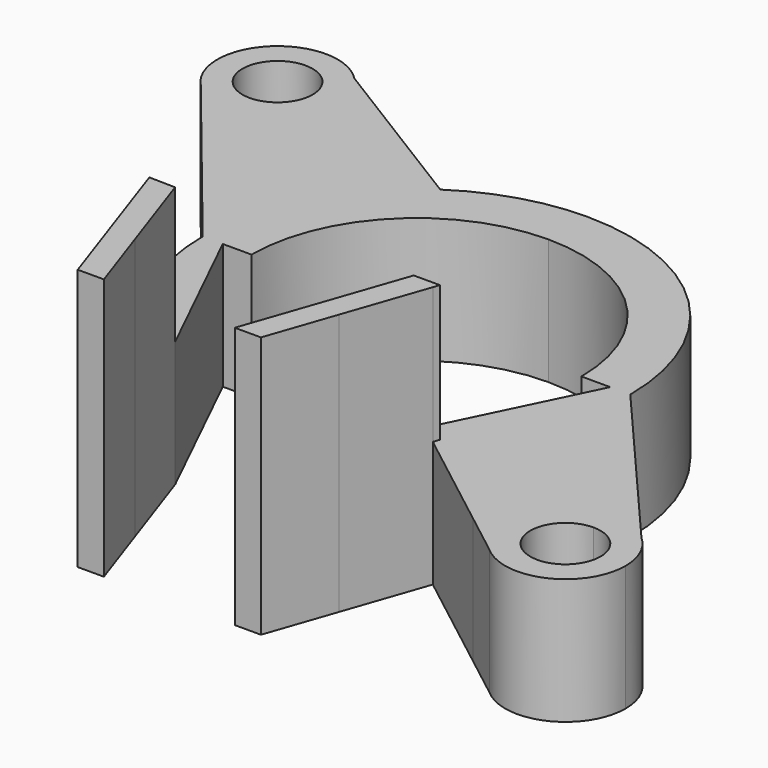
from build123d import *

# Parameters (mm, degrees)
F1_DEPTH = 12
F2_DEPTH = 25


# Not quite as in the source:
# - ends of sketch curves that miss each other by under 0.0002 mm in the source are joined


with BuildPart() as f1:
    # F0 (on Top) → F1 (new body)
    with BuildSketch(Plane.XY):
        with BuildLine():
            Line((-45.2079510631, 38.1848650801), (-50.0674114416, 38.1848649627))
            ThreePointArc((-50.0674114416, 38.1848649627), (-51.7515474497, 34.119000832), (-55.8174114415, 32.4348648238))
            Line((-55.8174114415, 32.4348648238), (-55.8174114414, 29.083605512))
            Line((-55.8174114414, 29.083605512), (-44.5532578407, 15.1687110318))
            ThreePointArc((-44.5532578407, 15.1687110318), (-42.1350647352, 24.8048651036), (-35.4555304308, 32.1592477879))
            Line((-35.4555304308, 32.1592477879), (-45.2079510631, 38.1848650801))
        make_face()
        with BuildLine():
            Line((-50.0674114416, 38.1848649627), (-52.4674114416, 38.1848649047))
            ThreePointArc((-52.4674114416, 38.1848649047), (-53.4486037246, 35.8160571069), (-55.8174114415, 34.8348648238))
            Line((-55.8174114415, 34.8348648238), (-55.8174114415, 32.4348648238))
            ThreePointArc((-55.8174114415, 32.4348648238), (-51.7515474497, 34.119000832), (-50.0674114416, 38.1848649627))
        make_face()
        with BuildLine():
            Line((-55.8174114414, 29.083605512), (-55.8174114415, 32.4348648238))
            ThreePointArc((-55.8174114415, 32.4348648238), (-58.0556968865, 32.8883963526), (-59.9408925855, 34.1774462962))
            Line((-59.9408925855, 34.1774462962), (-55.8174114414, 29.083605512))
        make_face()
        with BuildLine():
            Line((-55.8174114415, 32.4348648238), (-55.8174114415, 34.8348648238))
            ThreePointArc((-55.8174114415, 34.8348648238), (-57.1214560051, 35.0990962362), (-58.2197874124, 35.8501079425))
            Line((-58.2197874124, 35.8501079425), (-59.9408925855, 34.1774462962))
            ThreePointArc((-59.9408925855, 34.1774462962), (-58.0556968865, 32.8883963526), (-55.8174114415, 32.4348648238))
        make_face()
        with BuildLine():
            ThreePointArc((-58.2197874124, 35.8501079425), (-58.1521683229, 40.5872407946), (-53.4150354708, 40.5196217052))
            Line((-53.4150354708, 40.5196217052), (-51.6939302977, 42.1922833515))
            ThreePointArc((-51.6939302977, 42.1922833515), (-59.8248299692, 42.3083459677), (-59.9408925855, 34.1774462962))
            Line((-59.9408925855, 34.1774462962), (-58.2197874124, 35.8501079425))
        make_face()
        with BuildLine():
            ThreePointArc((-53.4150354708, 40.5196217052), (-52.7133447942, 39.4447339634), (-52.4674114416, 38.1848648238))
            Line((-52.4674114416, 38.1848648238), (-50.0674114416, 38.1848649627))
            ThreePointArc((-50.0674114416, 38.1848649627), (-50.4895358529, 40.3473267799), (-51.6939302977, 42.1922833515))
            Line((-51.6939302977, 42.1922833515), (-53.4150354708, 40.5196217052))
        make_face()
        with BuildLine():
            ThreePointArc((-51.6939302977, 42.1922833515), (-50.4895358529, 40.3473267799), (-50.0674114416, 38.1848648238))
            Line((-50.0674114416, 38.1848648238), (-45.2079510631, 38.1848650801))
            Line((-45.2079510631, 38.1848650801), (-51.6939302977, 42.1922833515))
        make_face()
        with BuildLine():
            ThreePointArc((-24.1338443596, 35.5853722206), (-30.0482104313, 34.7100811604), (-35.4555304308, 32.1592477879))
            ThreePointArc((-35.4555304308, 32.1592477879), (-42.1350647352, 24.8048651036), (-44.5532578407, 15.1687110318))
            Line((-44.5532578407, 15.1687110318), (-42.6338443592, 15.1659585535))
            Line((-42.6338443592, 15.1659585535), (-39.8838443592, 15.1659585535))
            ThreePointArc((-39.8838443592, 15.1659585535), (-35.270776163, 26.3028903571), (-24.1338443595, 30.9159585535))
            Line((-24.1338443595, 30.9159585535), (-24.1338443596, 35.5853722206))
        make_face()
        with BuildLine():
            ThreePointArc((-3.7144306922, 15.1659585535), (-9.6951384875, 29.6046644255), (-24.1338443596, 35.5853722206))
            Line((-24.1338443596, 35.5853722206), (-24.1338443595, 30.9159585535))
            ThreePointArc((-24.1338443595, 30.9159585535), (-12.9969125556, 26.3028903573), (-8.3838443592, 15.1659585535))
            Line((-8.3838443592, 15.1659585535), (-5.6338443592, 15.1659585535))
            Line((-5.6338443592, 15.1659585535), (-3.7144306922, 15.1659585535))
        make_face()
        with BuildLine():
            Line((-42.6338443592, 15.1659585535), (-44.5532578407, 15.1687110318))
            ThreePointArc((-44.5532578407, 15.1687110318), (-42.7914410163, 6.8685769492), (-37.807970261, 0.0011725238))
            Line((-37.807970261, 0.0011725238), (-38.0284454354, 0.643162408))
            Line((-38.0284454354, 0.643162408), (-35.5289696075, 0.5919707473))
            Line((-35.5289696075, 0.5919707473), (-42.6338443592, 15.1659585535))
        make_face()
        Polygon((-38.0284454354, 0.643162408), (-37.807970261, 0.0011725238), (-35.1236572441, -7.8151351762), (-32.6315665225, -7.8151351762), (-35.5289696075, 0.5919707473), align=None)
        Polygon((-32.6315665225, -7.8151351762), (-35.1236572441, -7.8151351762), (-32.8838443592, -14.3371266833), (-30.3838443592, -14.3371266833), align=None)
        Polygon((-13.136122196, -7.8151351762), (-15.636122196, -7.8151351762), (-17.8838443592, -14.3371266833), (-15.3838443592, -14.3371266833), align=None)
        Polygon((-10.2387191109, 0.5919707473), (-12.7387191109, 0.5919707473), (-15.636122196, -7.8151351762), (-13.136122196, -7.8151351762), (-10.4427343672, 0), align=None)
        with BuildLine():
            Line((7.5497227229, 2.079326472), (-3.7144306922, 15.1659585535))
            Line((-3.7144306922, 15.1659585535), (-5.6338443592, 15.1659585535))
            Line((-5.6338443592, 15.1659585535), (-12.7387191109, 0.5919707473))
            Line((-12.7387191109, 0.5919707473), (-10.2387191109, 0.5919707473))
            Line((-10.2387191109, 0.5919707473), (-10.4427343672, 0))
            Line((-10.4427343672, 0), (-0.3331204375, -7.8151351762))
            Line((-0.3331204375, -7.8151351762), (1.9170354556, -7.8151351762))
            ThreePointArc((1.9170354556, -7.8151351762), (3.0939956275, -3.0251503303), (7.549722723, -0.909568585))
            Line((7.549722723, -0.909568585), (7.5497227229, 2.079326472))
        make_face()
        with BuildLine():
            ThreePointArc((13.2997227231, -6.659568585), (12.7982725871, -4.3111171112), (11.3813838275, -2.3722765282))
            Line((11.3813838275, -2.3722765282), (9.7820818013, -4.1617549519))
            ThreePointArc((9.7820818013, -4.1617549519), (10.6075735134, -5.2913403351), (10.8997227231, -6.659568585))
            ThreePointArc((10.8997227231, -6.659568585), (8.917950973, -9.7174193754), (5.3173636448, -9.1573822181))
            Line((5.3173636448, -9.1573822181), (3.7180616186, -10.9468606418))
            ThreePointArc((3.7180616186, -10.9468606418), (9.8981741968, -11.908118449), (13.2997227231, -6.659568585))
        make_face()
        with BuildLine():
            ThreePointArc((11.3813838275, -2.3722765282), (9.6004019609, -1.2876774223), (7.549722723, -0.909568585))
            Line((7.549722723, -0.909568585), (7.549722723, -3.309568585))
            ThreePointArc((7.549722723, -3.309568585), (8.744466279, -3.5298580815), (9.7820818013, -4.1617549519))
            Line((9.7820818013, -4.1617549519), (11.3813838275, -2.3722765282))
        make_face()
        with BuildLine():
            Line((7.549722723, -3.309568585), (7.549722723, -0.909568585))
            ThreePointArc((7.549722723, -0.909568585), (3.0939956275, -3.0251503303), (1.9170354556, -7.8151351762))
            ThreePointArc((1.9170354556, -7.8151351762), (2.5652068364, -9.5261172721), (3.7180616186, -10.9468606418))
            Line((3.7180616186, -10.9468606418), (5.3173636448, -9.1573822181))
            ThreePointArc((5.3173636448, -9.1573822181), (4.4200122196, -5.464825029), (7.549722723, -3.309568585))
        make_face()
        with BuildLine():
            ThreePointArc((3.7180616186, -10.9468606418), (2.5652068364, -9.5261172721), (1.9170354556, -7.8151351762))
            Line((1.9170354556, -7.8151351762), (-0.3331204375, -7.8151351762))
            Line((-0.3331204375, -7.8151351762), (3.7180616186, -10.9468606418))
        make_face()
        with BuildLine():
            Line((11.3813838275, -2.3722765282), (7.5497227229, 2.079326472))
            Line((7.5497227229, 2.079326472), (7.549722723, -0.909568585))
            ThreePointArc((7.549722723, -0.909568585), (9.6004019609, -1.2876774223), (11.3813838275, -2.3722765282))
        make_face()
    extrude(amount=F1_DEPTH)

    # F0 (on Top) → F2 (join)
    with BuildSketch(Plane.XY):
        Polygon((-38.0284454354, 0.643162408), (-37.807970261, 0.0011725238), (-35.1236572441, -7.8151351762), (-32.6315665225, -7.8151351762), (-35.5289696075, 0.5919707473), align=None)
        Polygon((-32.6315665225, -7.8151351762), (-35.1236572441, -7.8151351762), (-32.8838443592, -14.3371266833), (-30.3838443592, -14.3371266833), align=None)
        Polygon((-13.136122196, -7.8151351762), (-15.636122196, -7.8151351762), (-17.8838443592, -14.3371266833), (-15.3838443592, -14.3371266833), align=None)
        Polygon((-10.2387191109, 0.5919707473), (-12.7387191109, 0.5919707473), (-15.636122196, -7.8151351762), (-13.136122196, -7.8151351762), (-10.4427343672, 0), align=None)
    extrude(amount=F2_DEPTH)


solid = f1.part
